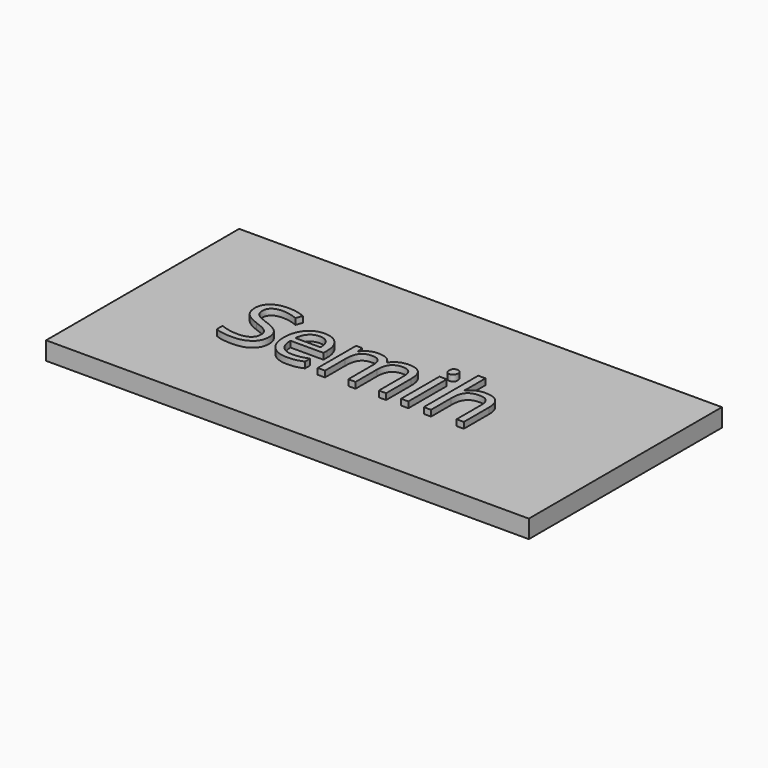
from build123d import *

# Parameters (mm, degrees)
F0_W         = 80
F0_H         = 40
F1_DEPTH     = 3
F2_TEXT_SIZE = 14.8518399025
F3_DEPTH     = 1


# Not quite as in the source:
# - Text() gives the source's letters only with a copy of the font that has no kerning and outlines rounded to 1/6400 em; it was checked with that copy


with BuildPart() as f1:
    # F0 (on Top) → F1 (new body)
    with BuildSketch(Plane.XY):
        with Locations((40, 20)):
            Rectangle(F0_W, F0_H)
    extrude(amount=F1_DEPTH)

    # F2 (on face) → F3 (join)
    with BuildSketch(Plane.XY.offset(3)):
        with Locations((15.7285481691, 14.4088026136)):
            Text('Semih', F2_TEXT_SIZE, font='Open Sans', text_align=(TextAlign.LEFT, TextAlign.BOTTOM))
    extrude(amount=F3_DEPTH)


solid = f1.part
